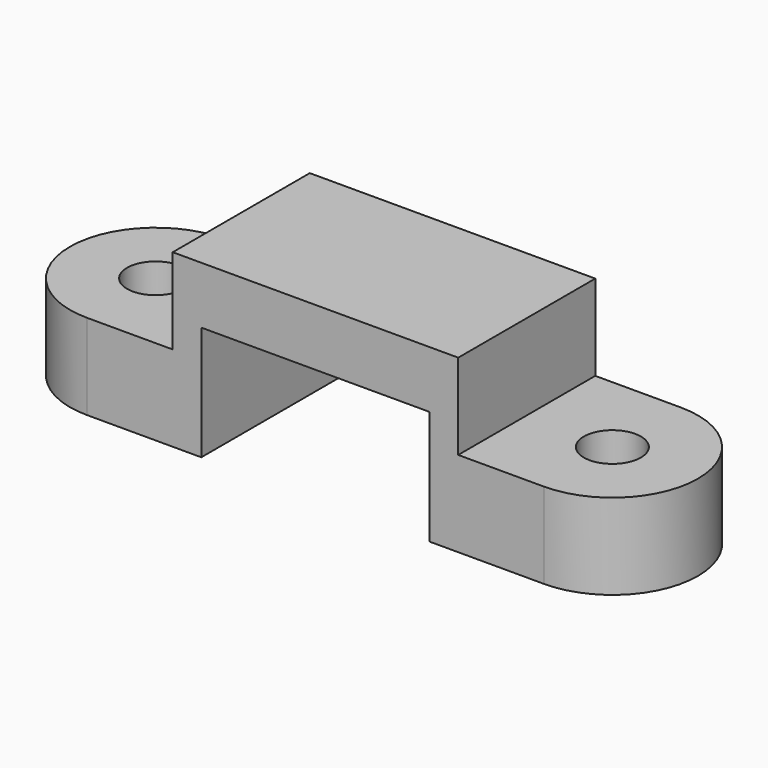
from build123d import *

# Parameters (mm, degrees)
F1_DEPTH = 9.525
F2_W     = 12.7
F2_H     = 9.525
F3_DEPTH = 6.35
F5_DEPTH = 4.7625
F7_R     = 1.5875
F6_R     = 1.5875
F8_DEPTH = 25.4


# Not quite as in the source:
# - a feature names something its author has since deleted; it is built from what else it names


with BuildPart() as f1:
    # F0 (on Top) → F1 (new body)
    with BuildSketch(Plane.XY):
        with BuildLine():
            ThreePointArc((0, 9.525), (-4.7625, 4.7625), (0, 0))
            Line((0, 0), (25.4, 0))
            ThreePointArc((25.4, 0), (30.1625, 4.7625), (25.4, 9.525))
            Line((25.4, 9.525), (0, 9.525))
        make_face()
    extrude(amount=F1_DEPTH)

    # F2 (on face) → F3 (cut)
    with BuildSketch(Plane(origin=(0, 0, 0), x_dir=(1, 0, 0), z_dir=(0, 0, -1))):
        with Locations((12.7, -4.7625)):
            Rectangle(F2_W, F2_H)
    extrude(amount=-F3_DEPTH, mode=Mode.SUBTRACT)

    # F4 (on face) → F5 (cut)
    with BuildSketch(Plane.XY.offset(9.525)):
        with BuildLine():
            Line((4.7625, 9.525), (0, 9.525))
            ThreePointArc((0, 9.525), (-4.7625, 4.7625), (0, 0))
            Line((0, 0), (4.7625, 0))
            Line((4.7625, 0), (4.7625, 9.525))
        make_face()
        with BuildLine():
            Line((25.4, 9.525), (20.6375, 9.525))
            Line((20.6375, 9.525), (20.6375, 0))
            Line((20.6375, 0), (25.4, 0))
            ThreePointArc((25.4, 0), (30.1625, 4.7625), (25.4, 9.525))
        make_face()
    extrude(amount=-F5_DEPTH, mode=Mode.SUBTRACT)

    # F7 (on face) + F6 (on face) → F8 (cut)
    with BuildSketch(Plane.XY.offset(4.7625)):
        with Locations((0, 4.7625)):
            Circle(F7_R)
    with BuildSketch(Plane.XY.offset(4.7625)):
        with Locations((25.4, 4.7625)):
            Circle(F6_R)
    extrude(amount=-F8_DEPTH, mode=Mode.SUBTRACT)


solid = f1.part
